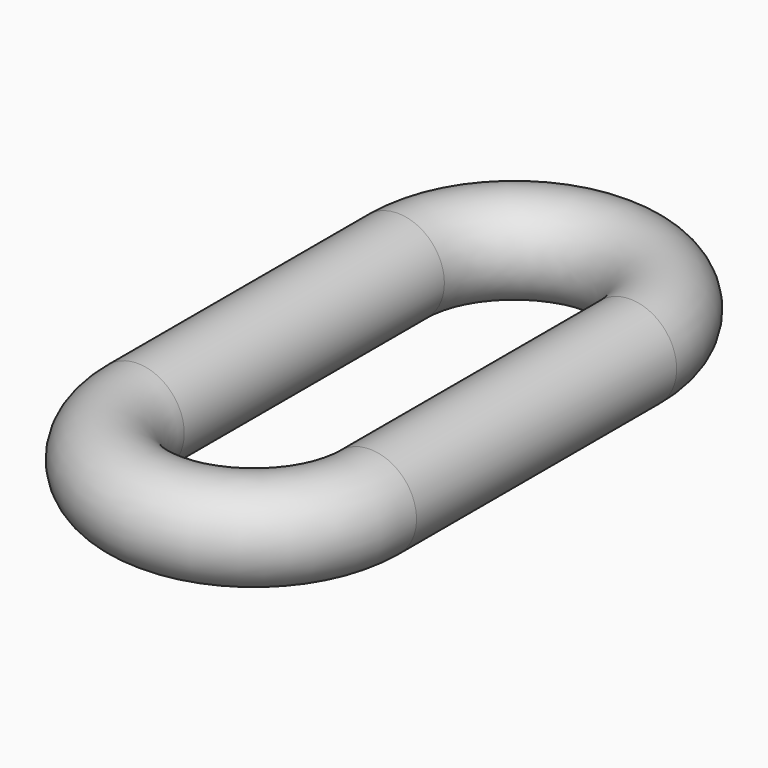
from build123d import *

# Parameters (mm, degrees)
F1_R = 1


# Not quite as in the source:
# - a feature of the source that left no trace in its solid (it failed there, or was rolled back) is left out


with BuildPart() as f2:
    # F2: sweep along a path in F0
    with BuildLine(Plane.XY) as f2_path:
        ThreePointArc((2.5, 3.5), (0, 6), (-2.5, 3.5))
        Line((-2.5, 3.5), (-2.5, -3.5))
        ThreePointArc((-2.5, -3.5), (0, -6), (2.5, -3.5))
        Line((2.5, -3.5), (2.5, 3.5))
    # F1 (on Front) → F2 (sweep)
    with BuildSketch(Plane.XZ):
        with Locations((-2.5, 0)):
            Circle(F1_R)
    sweep(path=f2_path.line)


solid = f2.part
